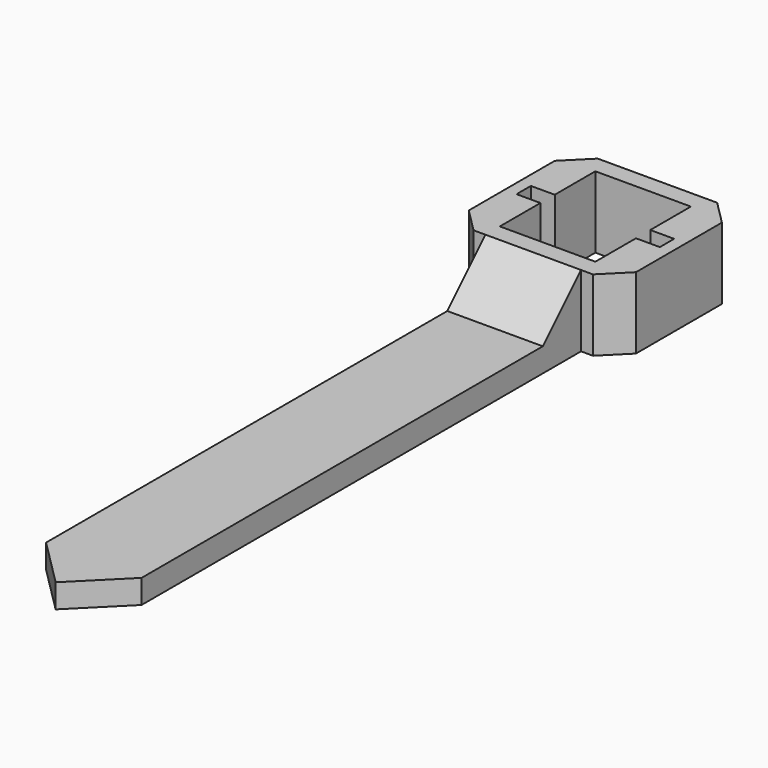
from build123d import *

# Parameters (mm, degrees)
F1_DEPTH = 6
F0_W     = 8
F0_H     = 50
F2_DEPTH = 2
F3_SIZE  = 3.99999
F4_SIZE  = 2


# Not quite as in the source:
# - a fillet or chamfer is up to 0.001 mm smaller than in the source, because OpenCascade refuses the exact size


with BuildPart() as f1:
    # F0 (on Top) → F1 (new body)
    with BuildSketch(Plane.XY):
        Polygon((4, -6.5), (7, -6.5), (7, 6.5), (-7, 6.5), (-7, -6.5), (-4, -6.5), align=None)
        Polygon((4, -0.75), (4, -5), (-4, -5), (-4, -0.75), (-6, -0.75), (-6, 0.75), (-4, 0.75), (-4, 5), (4, 5), (4, 0.75), (6, 0.75), (6, -0.75), align=None, mode=Mode.SUBTRACT)
    extrude(amount=F1_DEPTH)

    # F0 (on Top) → F2 (join)
    with BuildSketch(Plane.XY):
        with Locations((0, -31.5)):
            Rectangle(F0_W, F0_H)
    extrude(amount=F2_DEPTH)

    # F3 (size 4 in the source; OpenCascade refuses exactly that, so slightly less here)
    f3_edges = [f1.edges().sort_by_distance(p)[0] for p in [
        (0, -6.5, 2),
        (-4, -56.5, 1),
        (4, -56.5, 1),
    ]]
    chamfer(f3_edges, length=F3_SIZE)

    # F4
    f4_edges = [f1.edges().sort_by_distance(p)[0] for p in [
        (-7, -6.5, 3),
        (-7, 6.5, 3),
        (7, -6.5, 3),
        (7, 6.5, 3),
    ]]
    chamfer(f4_edges, length=F4_SIZE)


solid = f1.part
